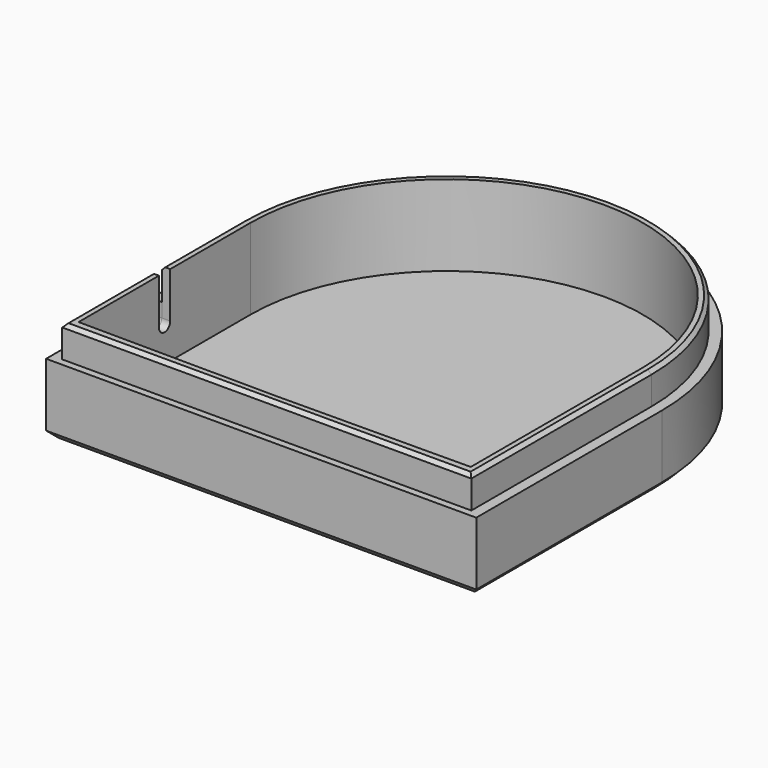
from build123d import *

# Parameters (mm, degrees)
F3_DEPTH  = 3
F4_DEPTH  = 10
F5_SIZE   = 0.99999
F8_DEPTH  = 11.5
F9_SIZE   = 0.5
F11_DEPTH = 25


# Not quite as in the source:
# - a fillet or chamfer is up to 0.001 mm smaller than in the source, because OpenCascade refuses the exact size
# - a feature of the source that left no trace in its solid (it failed there, or was rolled back) is left out
# - a feature names something its author has since deleted; it is built from what else it names


with BuildPart() as f3:
    # F2 (on Top) → F3 (new body)
    with BuildSketch(Plane.XY):
        with BuildLine():
            Line((29.1, -9.4630861774), (29.1, 0))
            ThreePointArc((29.1, 0), (0, -29.1), (-29.1, 0))
            Line((-29.1, 0), (-29.1, -9.4630861774))
            ThreePointArc((-29.1, -9.4630861774), (0, -30.6), (29.1, -9.4630861774))
        make_face()
        with BuildLine():
            ThreePointArc((-29.1, 0), (0, -29.1), (29.1, 0))
            Line((29.1, 0), (-29.1, 0))
        make_face()
        with BuildLine():
            Line((-29.1, 0), (29.1, 0))
            ThreePointArc((29.1, 0), (0, 29.1), (-29.1, 0))
        make_face()
        with BuildLine():
            Line((29.1, -32), (29.1, -9.4630861774))
            ThreePointArc((29.1, -9.4630861774), (0, -30.6), (-29.1, -9.4630861774))
            Line((-29.1, -9.4630861774), (-29.1, -32))
            Line((-29.1, -32), (29.1, -32))
        make_face()
    extrude(amount=F3_DEPTH)


with BuildPart() as f4:
    # F2 (on Top) → F4 (new body)
    with BuildSketch(Plane.XY):
        with BuildLine():
            ThreePointArc((30.6, 0), (30.2226736077, -4.7906158268), (29.1, -9.4630861774))
            Line((29.1, -9.4630861774), (29.1, -32))
            Line((29.1, -32), (-29.1, -32))
            Line((-29.1, -32), (-29.1, -9.4630861774))
            ThreePointArc((-29.1, -9.4630861774), (-30.2226736077, -4.7906158268), (-30.6, 0))
            Line((-30.6, 0), (-30.6, -33))
            Line((-30.6, -33), (30.6, -33))
            Line((30.6, -33), (30.6, 0))
        make_face()
        with BuildLine():
            ThreePointArc((-29.1, 0), (0, 29.1), (29.1, 0))
            Line((29.1, 0), (29.1, -9.4630861774))
            ThreePointArc((29.1, -9.4630861774), (30.2226736077, -4.7906158268), (30.6, 0))
            ThreePointArc((30.6, 0), (0, 30.6), (-30.6, 0))
            ThreePointArc((-30.6, 0), (-30.2226736077, -4.7906158268), (-29.1, -9.4630861774))
            Line((-29.1, -9.4630861774), (-29.1, 0))
        make_face()
    extrude(amount=F4_DEPTH)

    # F5 (size 1 in the source; OpenCascade refuses exactly that, so slightly less here)
    f5_edges = [f4.edges().sort_by_distance(p)[0] for p in [
        (30.6, -16.5, 0),
        (0, -33, 0),
        (-30.6, -16.5, 0),
        (0, 30.6, 0),
    ]]
    chamfer(f5_edges, length=F5_SIZE)


with BuildPart() as f8:
    # F6 (on face) → F8 (new body)
    with BuildSketch(Plane.XY.offset(3)):
        with BuildLine():
            Line((29.1, -32), (29.1, 0))
            ThreePointArc((29.1, 0), (0, 29.1), (-29.1, 0))
            Line((-29.1, 0), (-29.1, -32))
            Line((-29.1, -32), (29.1, -32))
        make_face()
        with BuildLine():
            ThreePointArc((-27.9, 0), (0, 27.9), (27.9, 0))
            Line((27.9, 0), (27.9, -30.6))
            Line((27.9, -30.6), (0, -30.7904947549))
            Line((0, -30.7904947549), (-27.9, -30.6))
            Line((-27.9, -30.6), (-27.9, 0))
        make_face(mode=Mode.SUBTRACT)
    extrude(amount=F8_DEPTH)

    # F9
    f9_edges = [f8.edges().sort_by_distance(p)[0] for p in [
        (-29.1, -16, 14.5),
        (0, 29.1, 14.5),
        (29.1, -16, 14.5),
        (0, -32, 14.5),
    ]]
    chamfer(f9_edges, length=F9_SIZE)


with BuildPart() as f11_tool:
    # F10 (on face) → F11 (new body)
    with BuildSketch(Plane.YZ.offset(-27.9)):
        with BuildLine():
            ThreePointArc((-16.3, 8), (-15.3, 7), (-14.3, 8))
            ThreePointArc((-14.3, 8), (-15.3, 9), (-16.3, 8))
        make_face()
        with BuildLine():
            ThreePointArc((-16.3, 8), (-15.3, 9), (-14.3, 8))
            Line((-14.3, 8), (-14.3, 14.5))
            Line((-14.3, 14.5), (-16.3, 14.5))
            Line((-16.3, 14.5), (-16.3, 8))
        make_face()
    extrude(amount=-F11_DEPTH)


with BuildPart() as f4_1:
    add(f4.part)

    # F11: cut by f11_tool
    add(f11_tool.part, mode=Mode.SUBTRACT)


with BuildPart() as f8_1:
    add(f8.part)

    # F11: cut by f11_tool
    add(f11_tool.part, mode=Mode.SUBTRACT)


solid = Compound([f3.part, f4_1.part, f8_1.part])
